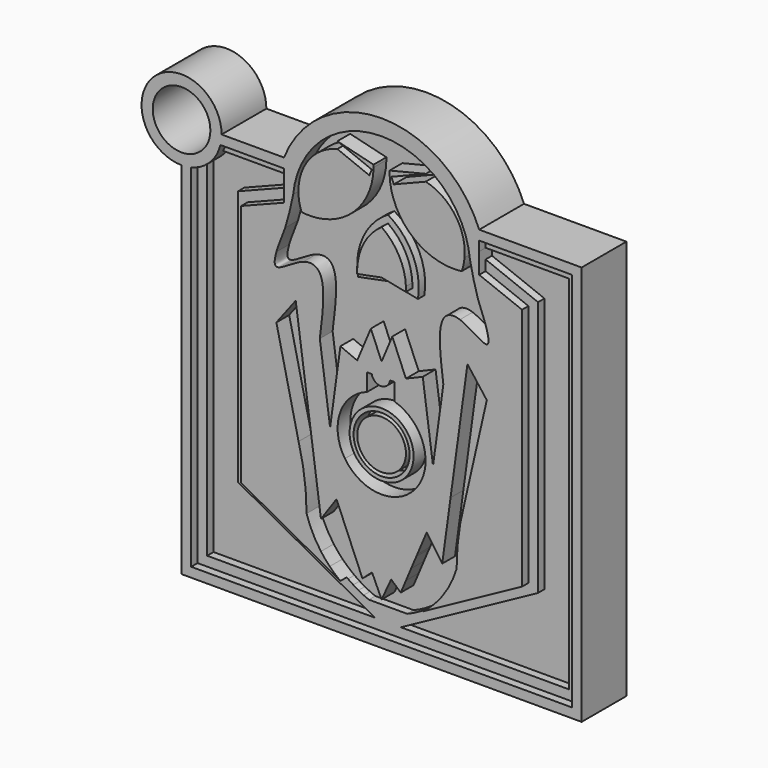
from build123d import *

# Parameters (mm, degrees)
F0_W      = 31.75
F0_H      = 31.75
F1_DEPTH  = 3.175
F3_DEPTH  = 1.27
F5_W      = 19.05
F5_H      = 4.445
F6_DEPTH  = 12.7
F4_R      = 2.54
F4_W      = 0.4114990976
F4_H      = 0.8219158335
F4_R_2    = 2.2225
F4_R_3    = 1.9327202177
F7_DEPTH  = 1.27
F9_DEPTH  = 1.27
F11_DEPTH = 1.27
F13_DEPTH = 25.4
F15_DEPTH = 0.635
F17_DEPTH = 0.635
F18_R     = 3.175
F19_DEPTH = 4.445
F20_R     = 2.286
F21_DEPTH = 25.4
F23_DEPTH = 0.635


# Not quite as in the source:
# - ends of sketch curves that miss each other by under 0.0002 mm in the source are joined


with BuildPart() as f1:
    # F0 (on Front) → F1 (new body)
    with BuildSketch(Plane.XZ):
        with Locations((15.875, 15.875)):
            Rectangle(F0_W, F0_H)
    extrude(amount=F1_DEPTH)

    # F2 (on face) → F3 (join)
    with BuildSketch(Plane.XZ.offset(3.175)):
        Polygon((0, 27.78125), (0, 0), (15.875, 0), (31.75, 0), (31.75, 31.75), (1.524, 31.75), (0, 31.75), align=None)
        Polygon((1.524, 1.524), (1.524, 30.226), (8.128, 30.226), (8.128, 29.4132), (3.96875, 27.78125), (3.96875, 7.46125), (14.859, 1.524), align=None, mode=Mode.SUBTRACT)
        Polygon((30.226, 30.226), (30.226, 1.524), (16.891, 1.524), (27.78125, 7.46125), (27.78125, 27.78125), (23.622, 29.4132), (23.622, 30.226), align=None, mode=Mode.SUBTRACT)
    extrude(amount=F3_DEPTH)

    # F5 (on face) → F6 (join)
    with BuildSketch(Plane.XY.offset(31.75)):
        with Locations((15.875, -2.2225)):
            Rectangle(F5_W, F5_H)
    extrude(amount=F6_DEPTH)

    # F4 (on face) → F7 (cut)
    with BuildSketch(Plane.XZ.offset(4.445)):
        Polygon((9.921875, 12.28725), (9.921875, 7.46125), (11.0631457555, 7.46125), (10.4008289927, 12.28725), align=None)
        with BuildLine():
            ThreePointArc((9.286875, 12.28725), (9.7624437739, 9.8950485229), (9.921875, 7.46125))
            Line((9.921875, 7.46125), (9.921875, 12.28725))
            Line((9.921875, 12.28725), (9.286875, 12.28725))
        make_face()
        with BuildLine():
            Line((11.0631457555, 7.46125), (9.921875, 7.46125))
            ThreePointArc((9.921875, 7.46125), (10.3968832716, 6.2759727233), (11.0631457555, 5.1866567071))
            Line((11.0631457555, 5.1866567071), (11.0631457555, 7.46125))
        make_face()
        Polygon((12.2976430482, 9.23925), (11.0631457555, 7.46125), (11.8861439507, 7.46125), (12.2976430482, 7.46125), align=None)
        Polygon((11.8861439507, 7.46125), (11.0631457555, 7.46125), (11.0631457555, 5.1866567071), (12.7091421458, 5.1866567071), (12.7091421458, 7.46125), (12.2976430482, 7.46125), align=None)
        Polygon((9.286875, 12.28725), (9.921875, 12.28725), (10.4008289927, 12.28725), (9.0599226916, 22.0578222886), (7.52475, 20.03425), align=None)
        with BuildLine():
            Line((12.7091421458, 5.1866567071), (11.0631457555, 5.1866567071))
            ThreePointArc((11.0631457555, 5.1866567071), (11.3972781469, 4.7633524228), (11.7605133391, 4.3647408736))
            Line((11.7605133391, 4.3647408736), (12.7091421458, 4.3647408736))
            Line((12.7091421458, 4.3647408736), (12.7091421458, 5.1866567071))
        make_face()
        Polygon((13.0481241495, 7.46125), (12.2976430482, 9.23925), (12.2976430482, 7.46125), (12.7091421458, 7.46125), align=None)
        with BuildLine():
            Line((12.7091421458, 4.3647408736), (11.7605133391, 4.3647408736))
            ThreePointArc((11.7605133391, 4.3647408736), (12.2178757018, 3.934217457), (12.7091421458, 3.5428250401))
            Line((12.7091421458, 3.5428250401), (12.7091421458, 4.3647408736))
        make_face()
        Polygon((12.7091421458, 7.46125), (12.7091421458, 5.1866567071), (12.7091421458, 4.3647408736), (13.1206412434, 4.3647408736), (13.1206412434, 7.2894463494), (13.0481241495, 7.46125), align=None)
        with BuildLine():
            Line((12.9632766086, 12.2909334156), (12.9646373774, 12.28725))
            Line((12.9646373774, 12.28725), (12.9657205058, 12.28725))
            ThreePointArc((12.9657205058, 12.28725), (12.9644979744, 12.2890913211), (12.9632766086, 12.2909334156))
        make_face()
        with BuildLine():
            Line((13.1206412434, 3.5311254517), (12.7091421458, 3.5428250401))
            ThreePointArc((12.7091421458, 3.5428250401), (12.9125963273, 3.3990611771), (13.1206412434, 3.2620248128))
            Line((13.1206412434, 3.2620248128), (13.1206412434, 3.5311254517))
        make_face()
        Polygon((12.7091421458, 4.3647408736), (12.7091421458, 3.5428250401), (13.1206412434, 3.5311254517), (13.1206412434, 4.3647408736), align=None)
        with BuildLine():
            ThreePointArc((12.9632766086, 12.2909334156), (12.9644979744, 12.2890913211), (12.9657205058, 12.28725))
            ThreePointArc((12.9657205058, 12.28725), (15.8746977849, 10.7274702177), (18.783675064, 12.28725))
            ThreePointArc((18.783675064, 12.28725), (18.7848975954, 12.2890913211), (18.7861189613, 12.2909334156))
            ThreePointArc((18.7861189613, 12.2909334156), (19.1648553848, 15.3914731915), (16.9118047418, 17.5549312984))
            Line((16.9118047418, 17.5549312984), (16.9118047418, 18.9191428908))
            Line((16.9118047418, 18.9191428908), (16.5426365201, 18.9191428908))
            ThreePointArc((16.5426365201, 18.9191428908), (15.8281814537, 18.2866264316), (15.0906208903, 18.8920416019))
            Line((15.0906208903, 18.8920416019), (14.7242317829, 18.8920416019))
            Line((14.7242317829, 18.8920416019), (14.7242317829, 17.5175426928))
            ThreePointArc((14.7242317829, 17.5175426928), (12.5650009715, 15.3350770527), (12.9632766086, 12.2909334156))
        make_face()
        with Locations((15.8746977849, 14.2199702177)):
            Circle(F4_R, mode=Mode.SUBTRACT)
        Polygon((13.532140341, 6.3145445242), (13.1206412434, 7.2894463494), (13.1206412434, 4.3647408736), (13.532140341, 4.3647408736), (13.532140341, 4.92125), align=None)
        with BuildLine():
            Line((13.1206412434, 3.5311254517), (13.1206412434, 3.2620248128))
            ThreePointArc((13.1206412434, 3.2620248128), (13.3244782061, 3.1369344232), (13.532140341, 3.0183024265))
            Line((13.532140341, 3.0183024265), (13.532140341, 3.5194258634))
            Line((13.532140341, 3.5194258634), (13.1206412434, 3.5311254517))
        make_face()
        Polygon((13.1206412434, 4.3647408736), (13.1206412434, 3.5311254517), (13.532140341, 3.5194258634), (13.532140341, 4.3647408736), align=None)
        with BuildLine():
            ThreePointArc((18.7861189613, 12.2909334156), (18.7848975954, 12.2890913211), (18.783675064, 12.28725))
            Line((18.783675064, 12.28725), (18.7853626226, 12.28725))
            Line((18.7853626226, 12.28725), (18.7861189613, 12.2909334156))
        make_face()
        Polygon((13.9436394385, 5.3396426989), (13.532140341, 6.3145445242), (13.532140341, 4.92125), (13.532140341, 4.3647408736), (13.9436394385, 4.3647408736), align=None)
        with BuildLine():
            Line((13.532140341, 3.5194258634), (13.532140341, 3.0183024265))
            ThreePointArc((13.532140341, 3.0183024265), (13.7362926994, 2.9098899022), (13.9436394385, 2.8077195021))
            Line((13.9436394385, 2.8077195021), (13.9436394385, 3.5077262751))
            Line((13.9436394385, 3.5077262751), (13.532140341, 3.5194258634))
        make_face()
        Polygon((13.532140341, 4.3647408736), (13.532140341, 3.5194258634), (13.9436394385, 3.5077262751), (13.9436394385, 4.3647408736), align=None)
        Polygon((14.3551385361, 4.3647408736), (13.9436394385, 5.3396426989), (13.9436394385, 4.3647408736), align=None)
        with BuildLine():
            Line((13.9436394385, 3.5077262751), (13.9436394385, 2.8077195021))
            ThreePointArc((13.9436394385, 2.8077195021), (14.1480589999, 2.7144823681), (14.3551385361, 2.6273125))
            Line((14.3551385361, 2.6273125), (14.3551385361, 3.4960266868))
            Line((14.3551385361, 3.4960266868), (13.9436394385, 3.5077262751))
        make_face()
        Polygon((13.9436394385, 4.3647408736), (13.9436394385, 3.5077262751), (14.3551385361, 3.4960266868), (14.3551385361, 4.3647408736), align=None)
        Polygon((21.828125, 12.28725), (21.3491710073, 12.28725), (20.6868542445, 7.46125), (21.828125, 7.46125), align=None)
        Polygon((22.6900773084, 22.0578222886), (21.3491710073, 12.28725), (21.828125, 12.28725), (22.463125, 12.28725), (24.22525, 20.03425), align=None)
        Polygon((15.115069268, 5.04428125), (14.3551385361, 4.3647408736), (14.3551385361, 3.4960266868), (14.3551385361, 2.6273125), (15.875, 2.6273125), (15.875, 3.3893125), align=None)
        Polygon((20.6868542445, 5.1866567071), (20.6868542445, 7.46125), (19.8638560493, 7.46125), (19.4523569518, 7.46125), (19.0408578542, 7.46125), (19.0408578542, 5.1866567071), align=None)
        with BuildLine():
            Line((21.828125, 7.46125), (20.6868542445, 7.46125))
            Line((20.6868542445, 7.46125), (20.6868542445, 5.1866567071))
            ThreePointArc((20.6868542445, 5.1866567071), (21.3531167284, 6.2759727233), (21.828125, 7.46125))
        make_face()
        Polygon((19.8638560493, 7.46125), (20.6868542445, 7.46125), (19.4523569518, 9.23925), (19.4523569518, 7.46125), align=None)
        with BuildLine():
            Line((22.463125, 12.28725), (21.828125, 12.28725))
            Line((21.828125, 12.28725), (21.828125, 7.46125))
            ThreePointArc((21.828125, 7.46125), (21.9875562261, 9.8950485229), (22.463125, 12.28725))
        make_face()
        Polygon((15.875, 3.3893125), (15.875, 2.6273125), (17.3948614639, 2.6273125), (17.3948614639, 3.5428250401), (17.3948614639, 4.3647408736), (16.634930732, 5.04428125), align=None)
        with BuildLine():
            ThreePointArc((19.9894866609, 4.3647408736), (20.3527218531, 4.7633524228), (20.6868542445, 5.1866567071))
            Line((20.6868542445, 5.1866567071), (19.0408578542, 5.1866567071))
            Line((19.0408578542, 5.1866567071), (19.0408578542, 4.3647408736))
            Line((19.0408578542, 4.3647408736), (19.9894866609, 4.3647408736))
        make_face()
        Polygon((19.4523569518, 7.46125), (19.4523569518, 9.23925), (18.7018758505, 7.46125), (19.0408578542, 7.46125), align=None)
        with BuildLine():
            Line((17.3948614639, 3.5428250401), (17.3948614639, 2.6273125))
            ThreePointArc((17.3948614639, 2.6273125), (17.6019410001, 2.7144823681), (17.8063605615, 2.8077195021))
            Line((17.8063605615, 2.8077195021), (17.8063605615, 3.5428250401))
            Line((17.8063605615, 3.5428250401), (17.3948614639, 3.5428250401))
        make_face()
        with BuildLine():
            ThreePointArc((19.0408578542, 3.5428250401), (19.5321242982, 3.934217457), (19.9894866609, 4.3647408736))
            Line((19.9894866609, 4.3647408736), (19.0408578542, 4.3647408736))
            Line((19.0408578542, 4.3647408736), (19.0408578542, 3.5428250401))
        make_face()
        Polygon((19.0408578542, 4.3647408736), (19.0408578542, 5.1866567071), (19.0408578542, 7.46125), (18.7018758505, 7.46125), (18.6293587566, 7.2894463494), (18.6293587566, 4.3647408736), align=None)
        with Locations((17.6006110127, 3.9537829568)):
            Rectangle(F4_W, F4_H)
        with BuildLine():
            Line((17.8063605615, 3.5428250401), (17.8063605615, 2.8077195021))
            ThreePointArc((17.8063605615, 2.8077195021), (18.0137073006, 2.9098899022), (18.217859659, 3.0183024265))
            Line((18.217859659, 3.0183024265), (18.217859659, 3.5428250401))
            Line((18.217859659, 3.5428250401), (17.8063605615, 3.5428250401))
        make_face()
        with Locations((18.8351083054, 3.9537829568)):
            Rectangle(F4_W, F4_H)
        with BuildLine():
            ThreePointArc((18.6293587566, 3.2620248128), (18.8374036727, 3.3990611771), (19.0408578542, 3.5428250401))
            Line((19.0408578542, 3.5428250401), (18.6293587566, 3.5428250401))
            Line((18.6293587566, 3.5428250401), (18.6293587566, 3.2620248128))
        make_face()
        Polygon((18.6293587566, 4.3647408736), (18.6293587566, 7.2894463494), (18.217859659, 6.3145445242), (18.217859659, 4.92125), (18.217859659, 4.3647408736), align=None)
        Polygon((17.8063605615, 5.3396426989), (17.3948614639, 4.3647408736), (17.8063605615, 4.3647408736), align=None)
        with Locations((18.0121101103, 3.9537829568)):
            Rectangle(F4_W, F4_H)
        with BuildLine():
            Line((18.217859659, 3.5428250401), (18.217859659, 3.0183024265))
            ThreePointArc((18.217859659, 3.0183024265), (18.4255217939, 3.1369344232), (18.6293587566, 3.2620248128))
            Line((18.6293587566, 3.2620248128), (18.6293587566, 3.5428250401))
            Line((18.6293587566, 3.5428250401), (18.217859659, 3.5428250401))
        make_face()
        with Locations((18.4236092078, 3.9537829568)):
            Rectangle(F4_W, F4_H)
        Polygon((18.217859659, 4.92125), (18.217859659, 6.3145445242), (17.8063605615, 5.3396426989), (17.8063605615, 4.3647408736), (18.217859659, 4.3647408736), align=None)
        with Locations((15.8746977849, 14.2199702177)):
            Circle(F4_R_2)
        with Locations((15.8746977849, 14.2199702177)):
            Circle(F4_R_3, mode=Mode.SUBTRACT)
        with BuildLine():
            Line((13.940829818, 19.4613496087), (15.0219064761, 22.0417031593))
            Line((15.0219064761, 22.0417031593), (15.8737911396, 20.0181308707))
            Line((15.8737911396, 20.0181308707), (16.7256758032, 22.0417031593))
            Line((16.7256758032, 22.0417031593), (17.8067555248, 19.4525339093))
            Line((17.8067555248, 19.4525339093), (19.1413669036, 20.0137266639))
            Line((19.1413669036, 20.0137266639), (19.9579843223, 14.057176314))
            Line((19.9579843223, 14.057176314), (20.7751547855, 20.0115245604))
            add(Edge.make_bspline(
                [(22.08911, 24.9660833333), (21.4903710735, 25.1745469914), (20.1770773703, 24.7924186118), (20.5393326656, 21.8811624654), (20.7751547855, 20.0115245604)],
                knots=[0.6284764605, 0.6284764605, 0.6284764605, 0.6284764605, 0.759913846, 1, 1, 1, 1], degree=3))
            Line((22.08911, 24.9660833333), (23.52675, 24.9660833333))
            Line((23.52675, 24.9660833333), (23.52675, 26.8710833333))
            Line((23.52675, 26.8710833333), (22.89175, 26.8710833333))
            Line((22.89175, 26.8710833333), (22.89175, 29.4110833333))
            ThreePointArc((22.89175, 29.4110833333), (22.6660820888, 30.6089193955), (22.2375120339, 31.75))
            Line((22.2375120339, 31.75), (15.875, 31.75))
            Line((15.875, 31.75), (9.5124879661, 31.75))
            ThreePointArc((9.5124879661, 31.75), (9.0839179112, 30.6089193955), (8.85825, 29.4110833333))
            Line((8.85825, 29.4110833333), (8.85825, 26.8710833333))
            Line((8.85825, 26.8710833333), (8.22325, 26.8710833333))
            Line((8.22325, 26.8710833333), (8.22325, 24.9660833333))
            Line((8.22325, 24.9660833333), (9.6609034253, 24.9660833333))
            add(Edge.make_bspline(
                [(9.6609034253, 24.9660833333), (10.2597091821, 25.1741950345), (11.5720822171, 24.7913696036), (11.2076515966, 21.8900971734), (10.9724274938, 20.0247371811)],
                knots=[0.6286821781, 0.6286821781, 0.6286821781, 0.6286821781, 0.7601673307, 1, 1, 1, 1], degree=3))
            Line((10.9724274938, 20.0247371811), (11.7899165807, 14.068067269))
            Line((11.7899165807, 14.068067269), (12.6062153757, 20.0225350776))
            Line((12.6062153757, 20.0225350776), (13.940829818, 19.4613496087))
        make_face()
        with BuildLine():
            add(Edge.make_bspline(
                [(7.52475, 24.9660833333), (7.391596508, 24.5029006383), (7.1808013336, 23.2509962569), (8.8732387699, 24.6923347437), (9.6609034253, 24.9660833333)],
                knots=[0.3416149305, 0.3416149305, 0.3416149305, 0.3416149305, 0.4557275825, 0.6286821781, 0.6286821781, 0.6286821781, 0.6286821781], degree=3))
            Line((9.6609034253, 24.9660833333), (8.22325, 24.9660833333))
            Line((8.22325, 24.9660833333), (7.52475, 24.9660833333))
        make_face()
        with BuildLine():
            add(Edge.make_bspline(
                [(8.22325, 26.8710833333), (7.9949590675, 26.1967451129), (7.7113735054, 25.6152647923), (7.52475, 24.9660833333)],
                knots=[0.1816784331, 0.1816784331, 0.1816784331, 0.1816784331, 0.3416149305, 0.3416149305, 0.3416149305, 0.3416149305], degree=3))
            Line((7.52475, 24.9660833333), (8.22325, 24.9660833333))
            Line((8.22325, 24.9660833333), (8.22325, 26.8710833333))
        make_face()
        with BuildLine():
            Line((23.52675, 24.9660833333), (22.08911, 24.9660833333))
            add(Edge.make_bspline(
                [(24.22525, 24.9660833333), (24.3584776917, 24.5026386829), (24.5693523519, 23.2495784284), (22.8766989585, 24.6918675307), (22.08911, 24.9660833333)],
                knots=[0.3414694731, 0.3414694731, 0.3414694731, 0.3414694731, 0.4555820168, 0.6284764605, 0.6284764605, 0.6284764605, 0.6284764605], degree=3))
            Line((24.22525, 24.9660833333), (23.52675, 24.9660833333))
        make_face()
        with BuildLine():
            add(Edge.make_bspline(
                [(8.85825, 29.4110833333), (8.6705499911, 28.52292058), (8.482575042, 27.6370918007), (8.22325, 26.8710833333)],
                knots=[0, 0, 0, 0, 0.1816784331, 0.1816784331, 0.1816784331, 0.1816784331], degree=3))
            Line((8.22325, 26.8710833333), (8.85825, 26.8710833333))
            Line((8.85825, 26.8710833333), (8.85825, 29.4110833333))
        make_face()
        with BuildLine():
            Line((23.52675, 26.8710833333), (23.52675, 24.9660833333))
            Line((23.52675, 24.9660833333), (24.22525, 24.9660833333))
            add(Edge.make_bspline(
                [(23.52675, 26.8710833333), (23.755024741, 26.1963929959), (24.0386018289, 25.6153559828), (24.22525, 24.9660833333)],
                knots=[0.1816010756, 0.1816010756, 0.1816010756, 0.1816010756, 0.3414694731, 0.3414694731, 0.3414694731, 0.3414694731], degree=3))
        make_face()
        with BuildLine():
            Line((22.89175, 26.8710833333), (23.52675, 26.8710833333))
            add(Edge.make_bspline(
                [(22.89175, 29.4110833333), (23.0794967523, 28.5247469343), (23.2674433506, 27.6374917849), (23.52675, 26.8710833333)],
                knots=[0, 0, 0, 0, 0.1816010756, 0.1816010756, 0.1816010756, 0.1816010756], degree=3))
            Line((22.89175, 29.4110833333), (22.89175, 26.8710833333))
        make_face()
        with BuildLine():
            ThreePointArc((15.875, 35.7610833333), (12.114336864, 34.674616256), (9.5124879661, 31.75))
            Line((9.5124879661, 31.75), (15.875, 31.75))
            Line((15.875, 31.75), (15.875, 35.7610833333))
        make_face()
        with BuildLine():
            ThreePointArc((22.2375120339, 31.75), (19.635663136, 34.674616256), (15.875, 35.7610833333))
            Line((15.875, 35.7610833333), (15.875, 31.75))
            Line((15.875, 31.75), (22.2375120339, 31.75))
        make_face()
    extrude(amount=-F7_DEPTH, mode=Mode.SUBTRACT)

    # F8 (on face) → F9 (join)
    with BuildSketch(Plane.XZ.offset(3.175)):
        with BuildLine():
            Line((13.940829818, 25.8887261599), (15.8737911396, 25.8887261599))
            Line((15.8737911396, 25.8887261599), (15.8737911396, 27.0628452177))
            Line((15.8737911396, 27.0628452177), (15.8737911396, 29.4110833333))
            ThreePointArc((15.8737911396, 29.4110833333), (14.4951241458, 27.8760999335), (13.940829818, 25.8887261599))
        make_face()
        Polygon((13.940829818, 25.5077261599), (15.8737911396, 25.8887261599), (13.940829818, 25.8887261599), align=None)
        with BuildLine():
            Line((15.8737911396, 27.0628452177), (15.8737911396, 25.8887261599))
            Line((15.8737911396, 25.8887261599), (17.8067555248, 25.8887261599))
            ThreePointArc((17.8067555248, 25.8887261599), (17.2524602507, 27.8761006132), (15.8737911396, 29.4110833333))
            Line((15.8737911396, 29.4110833333), (15.8737911396, 27.0628452177))
        make_face()
        Polygon((17.8067555248, 25.8887261599), (15.8737911396, 25.8887261599), (17.8067555248, 25.5077261599), align=None)
        with BuildLine():
            Line((13.940829818, 25.5077261599), (13.940829818, 25.8887261599))
            ThreePointArc((13.940829818, 25.8887261599), (13.9368198018, 25.6982261599), (13.940829818, 25.5077261599))
        make_face()
        with BuildLine():
            ThreePointArc((17.8067555248, 25.5077261599), (17.8107655447, 25.6982261599), (17.8067555248, 25.8887261599))
            Line((17.8067555248, 25.8887261599), (17.8067555248, 25.5077261599))
        make_face()
    extrude(amount=F9_DEPTH)

    # F10 (on face) → F11 (join)
    with BuildSketch(Plane.XZ.offset(3.175)):
        with BuildLine():
            Line((9.2902064724, 29.4110833333), (9.7351926425, 29.4110833333))
            Line((9.7351926425, 29.4110833333), (10.1736639637, 29.4110833333))
            Line((10.1736639637, 29.4110833333), (10.1736639637, 32.327852814))
            ThreePointArc((10.1736639637, 32.327852814), (9.4481700945, 30.9554174179), (9.2902064724, 29.4110833333))
        make_face()
        with BuildLine():
            Line((10.1736639637, 29.4110833333), (9.7351926425, 29.4110833333))
            Line((9.7351926425, 29.4110833333), (9.2902064724, 29.4110833333))
            ThreePointArc((9.2902064724, 29.4110833333), (9.370422983, 28.8958267112), (9.5159569818, 28.3950833333))
            Line((9.5159569818, 28.3950833333), (10.1736639637, 28.3950833333))
            Line((10.1736639637, 28.3950833333), (10.1736639637, 29.4110833333))
        make_face()
        with BuildLine():
            Line((10.1736639637, 32.327852814), (10.1736639637, 29.4110833333))
            Line((10.1736639637, 29.4110833333), (10.6121352849, 29.4110833333))
            Line((10.6121352849, 29.4110833333), (12.3660205698, 29.4110833333))
            Line((12.3660205698, 29.4110833333), (12.3660205698, 32.7074672028))
            Line((12.3660205698, 32.7074672028), (12.3660205698, 33.7234672028))
            ThreePointArc((12.3660205698, 33.7234672028), (11.155275335, 33.2056320492), (10.1736639637, 32.327852814))
        make_face()
        with BuildLine():
            Line((10.6121352849, 29.4110833333), (10.1736639637, 29.4110833333))
            Line((10.1736639637, 29.4110833333), (10.1736639637, 28.3950833333))
            Line((10.1736639637, 28.3950833333), (10.8029436449, 28.3950833333))
            ThreePointArc((10.8029436449, 28.3950833333), (12.0997831474, 28.7393237555), (13.2612620464, 29.4110833333))
            Line((13.2612620464, 29.4110833333), (12.3660205698, 29.4110833333))
            Line((12.3660205698, 29.4110833333), (10.6121352849, 29.4110833333))
        make_face()
        with BuildLine():
            Line((10.8029436449, 28.3950833333), (10.1736639637, 28.3950833333))
            Line((10.1736639637, 28.3950833333), (9.5159569818, 28.3950833333))
            ThreePointArc((9.5159569818, 28.3950833333), (10.1594503134, 28.3541622504), (10.8029436449, 28.3950833333))
        make_face()
        with BuildLine():
            Line((12.3660205698, 32.7074672028), (12.3660205698, 29.4110833333))
            Line((12.3660205698, 29.4110833333), (13.2612620464, 29.4110833333))
            ThreePointArc((13.2612620464, 29.4110833333), (14.7037114788, 31.1634596146), (15.2390338372, 33.3691143856))
            Line((15.2390338372, 33.3691143856), (15.239110373, 33.5684491949))
            Line((15.239110373, 33.5684491949), (12.3660205698, 34.2705999472))
            Line((12.3660205698, 34.2705999472), (13.4425796787, 33.8399763036))
            Line((13.4425796787, 33.8399763036), (15.0946870334, 33.1791333618))
            Line((15.0946870334, 33.1791333618), (14.9060205698, 32.7074672028))
            Line((14.9060205698, 32.7074672028), (12.3660205698, 32.7074672028))
        make_face()
        Polygon((14.9060205698, 32.7074672028), (12.3660205698, 33.7234672028), (12.3660205698, 32.7074672028), align=None)
        with BuildLine():
            ThreePointArc((22.89175, 29.4110833333), (22.4705122339, 31.2432868308), (21.5758827137, 32.8967828039))
            Line((21.5758827137, 32.8967828039), (21.5758827137, 32.8598922996))
            ThreePointArc((21.5758827137, 32.8598922996), (22.4634836102, 31.2231156406), (22.89175, 29.4110833333))
        make_face()
        with BuildLine():
            Line((16.5087911396, 33.5683516994), (16.5087911396, 33.3690168842))
            ThreePointArc((16.5087911396, 33.3690168842), (17.0439904781, 31.1634607611), (18.4862420146, 29.4110833333))
            Line((18.4862420146, 29.4110833333), (19.3827705698, 29.4110833333))
            Line((19.3827705698, 29.4110833333), (19.3827705698, 32.7089682218))
            Line((19.3827705698, 32.7089682218), (16.8427705698, 32.7089682218))
            Line((16.8427705698, 32.7089682218), (16.6541041062, 33.1806343807))
            Line((16.6541041062, 33.1806343807), (18.3051918751, 33.8410694883))
            Line((18.3051918751, 33.8410694883), (19.3827705698, 34.2721009662))
            Line((19.3827705698, 34.2721009662), (16.5087911396, 33.5683516994))
        make_face()
        with BuildLine():
            ThreePointArc((22.2338163568, 28.3950833333), (22.3795093305, 28.8958161501), (22.4598805081, 29.4110833333))
            Line((22.4598805081, 29.4110833333), (22.0145051425, 29.4110833333))
            Line((22.0145051425, 29.4110833333), (21.5758827137, 29.4110833333))
            Line((21.5758827137, 29.4110833333), (21.5758827137, 28.3950833333))
            Line((21.5758827137, 28.3950833333), (22.2338163568, 28.3950833333))
        make_face()
        with BuildLine():
            Line((22.0145051425, 29.4110833333), (22.4598805081, 29.4110833333))
            ThreePointArc((22.4598805081, 29.4110833333), (22.302041026, 30.9565099921), (21.5758827137, 32.3298092912))
            Line((21.5758827137, 32.3298092912), (21.5758827137, 29.4110833333))
            Line((21.5758827137, 29.4110833333), (22.0145051425, 29.4110833333))
        make_face()
        with BuildLine():
            Line((21.5758827137, 29.4110833333), (21.5758827137, 32.3298092912))
            ThreePointArc((21.5758827137, 32.3298092912), (20.5938744584, 33.2074515453), (19.3827705698, 33.7249682218))
            Line((19.3827705698, 33.7249682218), (19.3827705698, 32.7089682218))
            Line((19.3827705698, 32.7089682218), (19.3827705698, 29.4110833333))
            Line((19.3827705698, 29.4110833333), (21.1372602849, 29.4110833333))
            Line((21.1372602849, 29.4110833333), (21.5758827137, 29.4110833333))
        make_face()
        with BuildLine():
            Line((19.3827705698, 29.4110833333), (18.4862420146, 29.4110833333))
            ThreePointArc((18.4862420146, 29.4110833333), (19.646948682, 28.7395275515), (20.9429368441, 28.3950833333))
            Line((20.9429368441, 28.3950833333), (21.5758827137, 28.3950833333))
            Line((21.5758827137, 28.3950833333), (21.5758827137, 29.4110833333))
            Line((21.5758827137, 29.4110833333), (21.1372602849, 29.4110833333))
            Line((21.1372602849, 29.4110833333), (19.3827705698, 29.4110833333))
        make_face()
        with BuildLine():
            ThreePointArc((20.9429368441, 28.3950833333), (21.5883766005, 28.3539133087), (22.2338163568, 28.3950833333))
            Line((22.2338163568, 28.3950833333), (21.5758827137, 28.3950833333))
            Line((21.5758827137, 28.3950833333), (20.9429368441, 28.3950833333))
        make_face()
        Polygon((19.3827705698, 32.7089682218), (19.3827705698, 33.7249682218), (16.8427705698, 32.7089682218), align=None)
    extrude(amount=F11_DEPTH)

    # F12 (on face) → F13 (cut)
    with BuildSketch(Plane.XZ.offset(4.445)):
        with BuildLine():
            Line((6.35, 44.45), (6.35, 31.75))
            Line((6.35, 31.75), (8.1271030349, 31.75))
            ThreePointArc((8.1271030349, 31.75), (15.875, 37.0186869701), (23.6228969651, 31.75))
            Line((23.6228969651, 31.75), (25.4, 31.75))
            Line((25.4, 31.75), (25.4, 44.45))
            Line((25.4, 44.45), (6.35, 44.45))
        make_face()
    extrude(amount=-F13_DEPTH, mode=Mode.SUBTRACT)

    # F14 (on face) → F15 (cut)
    with BuildSketch(Plane.XZ.offset(4.445)):
        Polygon((8.1275515175, 30.988), (0.762, 30.988), (1.524, 30.226), (8.128, 30.226), align=None)
        Polygon((1.524, 30.226), (0.762, 30.988), (0.762, 0.762), (30.988, 0.762), (30.988, 30.988), (23.6224484825, 30.988), (23.622, 30.226), (30.226, 30.226), (30.226, 1.524), (16.891, 1.524), (14.859, 1.524), (1.524, 1.524), align=None)
    extrude(amount=-F15_DEPTH, mode=Mode.SUBTRACT)

    # F16 (on face) → F17 (cut)
    with BuildSketch(Plane.XZ.offset(4.445)):
        with BuildLine():
            Line((8.128, 28.5946433694), (8.128, 29.4132))
            Line((8.128, 29.4132), (3.96875, 27.78125))
            Line((3.96875, 27.78125), (3.96875, 7.46125))
            Line((3.96875, 7.46125), (14.859, 1.524))
            Line((14.859, 1.524), (16.891, 1.524))
            Line((16.891, 1.524), (27.78125, 7.46125))
            Line((27.78125, 7.46125), (27.78125, 27.78125))
            Line((27.78125, 27.78125), (23.622, 29.4132))
            Line((23.622, 29.4132), (23.622, 28.5946433694))
            Line((23.622, 28.5946433694), (27.01925, 27.2616765755))
            Line((27.01925, 27.2616765755), (27.01925, 7.9137036911))
            Line((27.01925, 7.9137036911), (19.1467784676, 3.6217148381))
            ThreePointArc((19.1467784676, 3.6217148381), (18.3029608199, 3.067888592), (17.3948614639, 2.6273125))
            Line((17.3948614639, 2.6273125), (17.3228212378, 2.6273125))
            Line((17.3228212378, 2.6273125), (14.4271787622, 2.6273125))
            Line((14.4271787622, 2.6273125), (14.3551385361, 2.6273125))
            ThreePointArc((14.3551385361, 2.6273125), (13.4470391801, 3.067888592), (12.6032215324, 3.6217148381))
            Line((12.6032215324, 3.6217148381), (4.73075, 7.9137036911))
            Line((4.73075, 7.9137036911), (4.73075, 27.2616765755))
            Line((4.73075, 27.2616765755), (8.128, 28.5946433694))
        make_face()
    extrude(amount=-F17_DEPTH, mode=Mode.SUBTRACT)

    # F18 (on face) → F19 (join)
    with BuildSketch(Plane.XZ.offset(4.445)):
        with Locations((0, 31.75)):
            Circle(F18_R)
    extrude(amount=-F19_DEPTH)

    # F20 (on face) → F21 (cut)
    with BuildSketch(Plane.XZ.offset(4.445)):
        with Locations((0, 31.75)):
            Circle(F20_R)
    extrude(amount=-F21_DEPTH, mode=Mode.SUBTRACT)

    # F22 (on face) → F23 (join)
    with BuildSketch(Plane.XZ.offset(3.175)):
        with BuildLine():
            ThreePointArc((18.2553347761, 24.9015341117), (17.8481736582, 27.82363386), (15.8737907374, 30.0159520846))
            ThreePointArc((15.8737907374, 30.0159520846), (13.8994107299, 27.8236327099), (13.4922505461, 24.9015339368))
            Line((13.4922505461, 24.9015339368), (15.8737912175, 25.3709520186))
            Line((15.8737912175, 25.3709520186), (18.2553347761, 24.9015341117))
        make_face()
    extrude(amount=F23_DEPTH)


solid = f1.part
